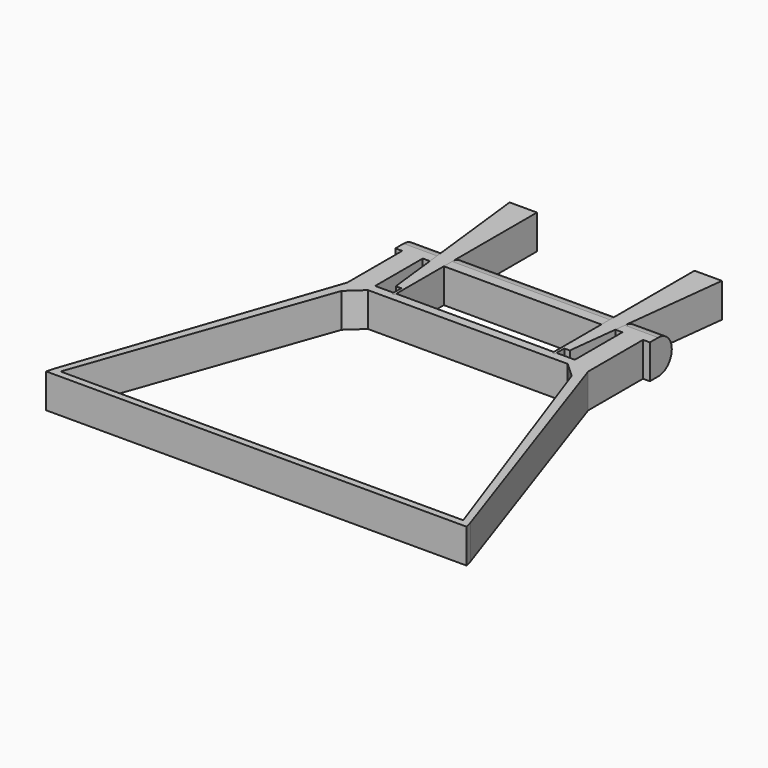
from build123d import *

# Parameters (mm, degrees)
F0_W     = 145.8
F0_H     = 6.5740418434
F1_DEPTH = 25
F2_W     = 2
F2_H     = 8.6666666667
F3_DEPTH = 25
F4_R     = 12.4


# Not quite as in the source:
# - a feature names something its author has since deleted; it is built from what else it names


with BuildPart() as f1:
    # F0 (on Top) → F1 (new body)
    with BuildSketch(Plane.XY):
        Polygon((153.4961182735, -262.9485861983), (152.1440880223, -257.9410667492), (87.9, -70), (87.9, -20), (92.9, -20), (92.9, 0), (88.236759305, 0), (-88.236759305, 0), (-92.9, 0), (-92.9, -20), (-87.9, -20), (-87.9, -70), (-152.1440880223, -257.9410667492), (-153.4961182735, -262.9485861983), align=None)
        Polygon((83.9809148248, -80.1100606648), (146.9573287566, -257.9124928518), (-146.9573287566, -257.9124928518), (-83.9809148248, -80.1100606648), (-72.9, -70), (-72.9, -63.4259581566), (-72.9, -20), (72.9, -20), (72.9, -63.4259581566), (72.9, -70), align=None, mode=Mode.SUBTRACT)
        with Locations((0, -66.7129790783)):
            Rectangle(F0_W, F0_H)
    extrude(amount=F1_DEPTH)

    # F4
    f4_edges = [f1.edges().sort_by_distance(p)[0] for p in [
        (0, 0, 25),
        (0, 0, 0),
    ]]
    fillet(f4_edges, radius=F4_R)


with BuildPart() as f3:
    # F2 (on Top) → F3 (new body)
    with BuildSketch(Plane.XY):
        Polygon((-57.5, -56.3333333333), (-57.5, 0), (-57.5, 65), (-77.5, 65), (-63.5, -56.3333333333), (-59.5, -56.3333333333), align=None)
        with Locations((-58.5, -60.6666666667)):
            Rectangle(F2_W, F2_H)
    extrude(amount=F3_DEPTH)


with BuildPart() as f3b:
    # F2 (on Top) → F3, piece 2 (new body)
    with BuildSketch(Plane.XY):
        Polygon((57.5, 65), (57.5, 0), (57.5, -56.3333333333), (59.5, -56.3333333333), (63.5, -56.3333333333), (77.5, 65), align=None)
        with Locations((58.5, -60.6666666667)):
            Rectangle(F2_W, F2_H)
    extrude(amount=F3_DEPTH)


solid = Compound([f1.part, f3.part, f3b.part])
